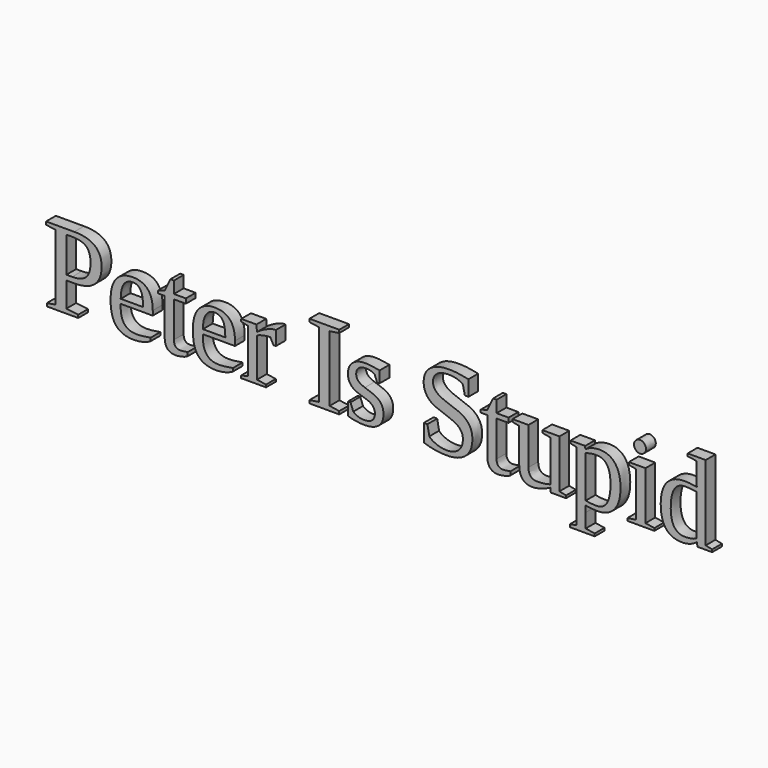
from build123d import *

# Parameters (mm, degrees)
F0_TEXT_SIZE = 237.1839765045
F1_DEPTH     = 25.4


# Not quite as in the source:
# - Text() gives the source's letters only with a copy of the font that has no kerning and outlines rounded to 1/6400 em; it was checked with that copy


with BuildPart() as f1:
    # F0 (on Front) → F1 (new body)
    with BuildSketch(Plane.XZ):
        with Locations((-153.0669480562, -85.1006582379)):
            Text('Peter Is Stupid', F0_TEXT_SIZE, font='Tinos', text_align=(TextAlign.LEFT, TextAlign.BOTTOM))
    extrude(amount=F1_DEPTH)


solid = f1.part
